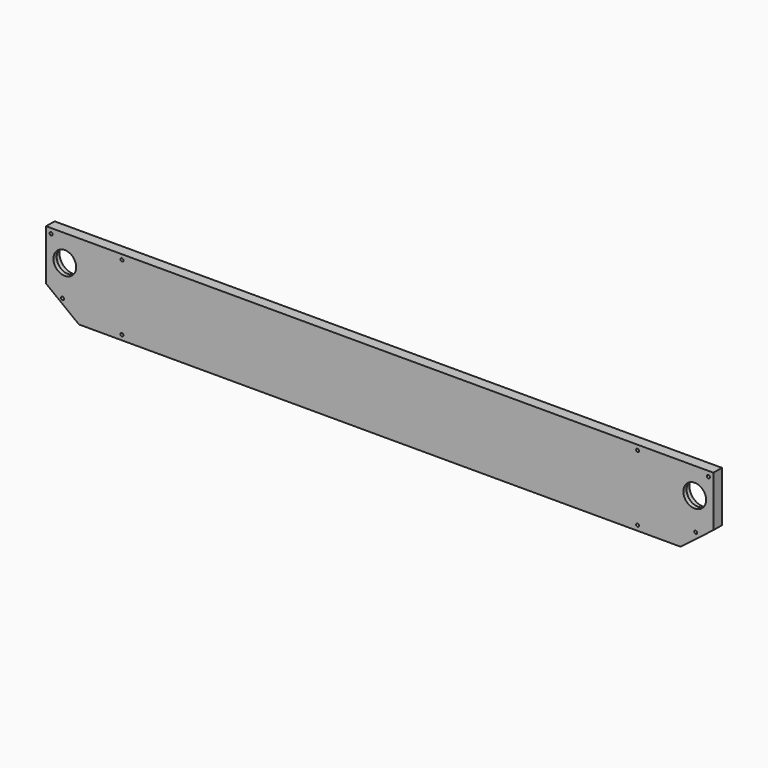
from build123d import *

# Parameters (mm, degrees)
F0_R     = 3
F0_R_2   = 27.5
F1_DEPTH = 21
F2_R     = 27.5
F2_R_2   = 22.5
F3_DEPTH = 8


# Not quite as in the source:
# - a feature names something its author has since deleted; it is built from what else it names


with BuildPart() as f1:
    # F0 (on Front) → F1 (new body)
    with BuildSketch(Plane.XZ):
        Polygon((0, 50), (65, 0), (160, 0), (1255.0009576903, 0), (1320, 50), (1320, 150), (160, 150), (0, 150), (0, 120), align=None)
        with Locations((150, 10)):
            Circle(F0_R, mode=Mode.SUBTRACT)
        with Locations((32.5, 35)):
            Circle(F0_R, mode=Mode.SUBTRACT)
        with Locations((1170, 10)):
            Circle(F0_R, mode=Mode.SUBTRACT)
        with Locations((1285, 35)):
            Circle(F0_R, mode=Mode.SUBTRACT)
        with Locations((37, 98)):
            Circle(F0_R_2, mode=Mode.SUBTRACT)
        with Locations((10, 140)):
            Circle(F0_R, mode=Mode.SUBTRACT)
        with Locations((150, 140)):
            Circle(F0_R, mode=Mode.SUBTRACT)
        with Locations((1283, 98)):
            Circle(F0_R_2, mode=Mode.SUBTRACT)
        with Locations((1170, 140)):
            Circle(F0_R, mode=Mode.SUBTRACT)
        with Locations((1310, 140)):
            Circle(F0_R, mode=Mode.SUBTRACT)
    extrude(amount=-F1_DEPTH)

    # F2 (on face) → F3 (join)
    with BuildSketch(Plane.XZ):
        with Locations((1283, 98)):
            Circle(F2_R)
        with Locations((1283, 98)):
            Circle(F2_R_2, mode=Mode.SUBTRACT)
        with Locations((37, 98)):
            Circle(F2_R)
        with Locations((37, 98)):
            Circle(F2_R_2, mode=Mode.SUBTRACT)
    extrude(amount=-F3_DEPTH)


solid = f1.part
